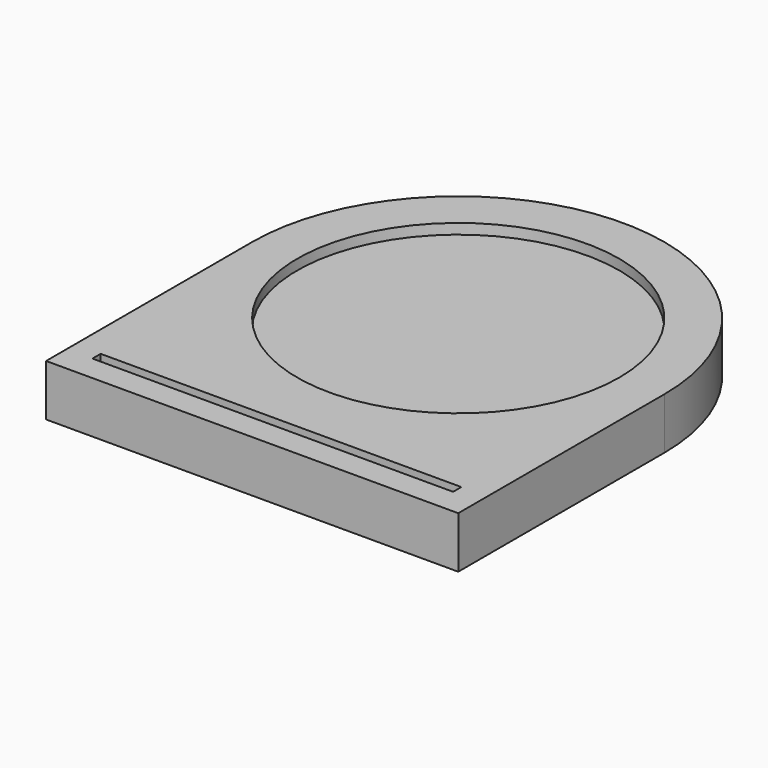
from build123d import *

# Parameters (mm, degrees)
F1_DEPTH = 20
F2_R     = 62.5
F3_DEPTH = 4
F4_W     = 140
F4_H     = 4
F5_DEPTH = 12


# Not quite as in the source:
# - a feature of the source that left no trace in its solid (it failed there, or was rolled back) is left out


with BuildPart() as f1:
    # F0 (on Top) → F1 (new body)
    with BuildSketch(Plane.XY):
        with BuildLine():
            Line((80, -100), (80, 0))
            ThreePointArc((80, 0), (0, 80), (-80, 0))
            Line((-80, 0), (-80, -100))
            Line((-80, -100), (80, -100))
        make_face()
    extrude(amount=F1_DEPTH)

    # F2 (on face) → F3 (cut)
    with BuildSketch(Plane.XY.offset(20)):
        Circle(F2_R)
    extrude(amount=-F3_DEPTH, mode=Mode.SUBTRACT)

    # F4 (on face) → F5 (cut)
    with BuildSketch(Plane.XY.offset(20)):
        with Locations((0, -88)):
            Rectangle(F4_W, F4_H)
    extrude(amount=-F5_DEPTH, mode=Mode.SUBTRACT)


solid = f1.part
